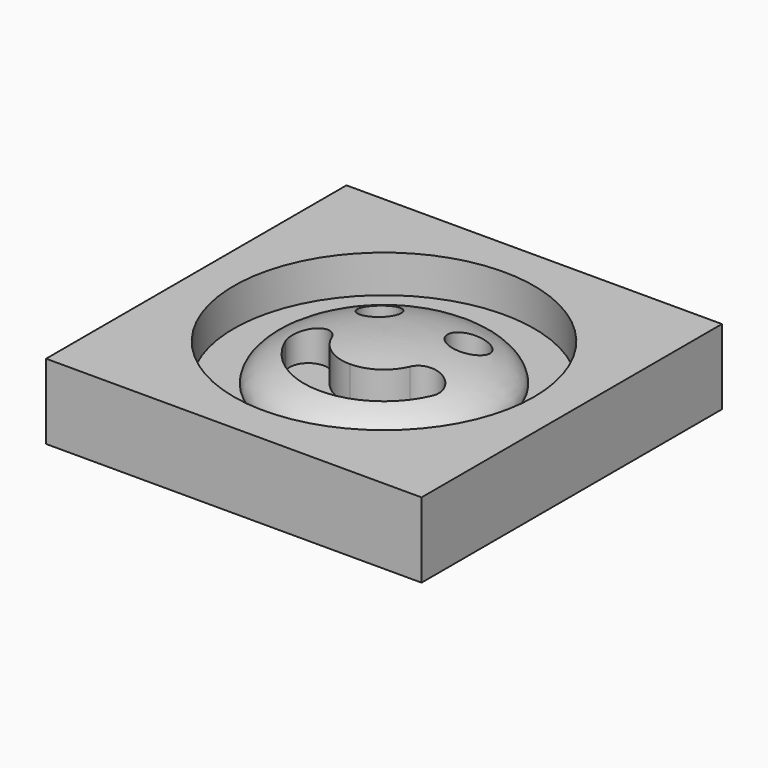
from build123d import *

# Parameters (mm, degrees)
F2_R     = 2.5
F3_DEPTH = 25
F4_R     = 20
F4_R_2   = 15
F4_R_3   = 2.5
F5_DEPTH = 5
F6_DEPTH = 5


with BuildPart() as f1:
    # F0 (on Front) → F1 (revolve)
    with BuildSketch(Plane.XZ):
        with BuildLine():
            Line((0, 0), (0, 5))
            add(Edge.make_bspline(
                [(0, 5), (-15, 5), (-15, 0)],
                knots=[4.7123889804, 4.7123889804, 4.7123889804, 6.2831853072, 6.2831853072, 6.2831853072], degree=2, weights=[1, 0.7071067812, 1]))
            Line((-15, 0), (0, 0))
        make_face()
    revolve(axis=Axis((0, 0, 2.5), (0, 0, 1)))

    # F2 (on face) → F3 (cut)
    with BuildSketch(Plane(origin=(0, 0, 0), x_dir=(1, 0, 0), z_dir=(0, 0, -1))):
        with Locations((5.9301354922, -6.6626928747)):
            Circle(F2_R)
        with BuildLine():
            ThreePointArc((-5.2131647244, 2.2031189874), (-3.1274667568, 4.7169663346), (0, 5.6595776977))
            ThreePointArc((0, 5.6595776977), (3.1274667568, 4.7169663346), (5.2131647244, 2.2031189874))
            ThreePointArc((5.2131647244, 2.2031189874), (8.4891528404, 0.8734942796), (9.8187775482, 4.1494823956))
            ThreePointArc((9.8187775482, 4.1494823956), (5.8904527284, 8.8842086506), (0, 10.6595776977))
            ThreePointArc((0, 10.6595776977), (-5.8904527284, 8.8842086506), (-9.8187775482, 4.1494823956))
            ThreePointArc((-9.8187775482, 4.1494823956), (-8.4891528404, 0.8734942796), (-5.2131647244, 2.2031189874))
        make_face()
        with Locations((-5.9301354922, -6.6626928747)):
            Circle(F2_R)
    extrude(amount=-F3_DEPTH, mode=Mode.SUBTRACT)

    # F4 (on face) → F5 (join)
    with BuildSketch(Plane(origin=(0, 0, 0), x_dir=(1, 0, 0), z_dir=(0, 0, -1))):
        Polygon((-25, -25), (0, -25), (25, -25), (25, 0), (25, 25), (0, 25), (-25, 25), (-25, 0), align=None)
        Circle(F4_R, mode=Mode.SUBTRACT)
        Circle(F4_R)
        Circle(F4_R_2, mode=Mode.SUBTRACT)
        Circle(F4_R_2)
        with Locations((-5.9301354922, -6.6626928747)):
            Circle(F4_R_3, mode=Mode.SUBTRACT)
        with Locations((5.9301354922, -6.6626928747)):
            Circle(F4_R_3, mode=Mode.SUBTRACT)
        with BuildLine():
            ThreePointArc((-5.2131647244, 2.2031189874), (-8.4891528404, 0.8734942796), (-9.8187775482, 4.1494823956))
            ThreePointArc((-9.8187775482, 4.1494823956), (0, 10.6595776977), (9.8187775482, 4.1494823956))
            ThreePointArc((9.8187775482, 4.1494823956), (8.4891528404, 0.8734942796), (5.2131647244, 2.2031189874))
            ThreePointArc((5.2131647244, 2.2031189874), (0, 5.6595776977), (-5.2131647244, 2.2031189874))
        make_face(mode=Mode.SUBTRACT)
        with BuildLine():
            ThreePointArc((9.8187775482, 4.1494823956), (0, 10.6595776977), (-9.8187775482, 4.1494823956))
            ThreePointArc((-9.8187775482, 4.1494823956), (-8.4891528404, 0.8734942796), (-5.2131647244, 2.2031189874))
            ThreePointArc((-5.2131647244, 2.2031189874), (0, 5.6595776977), (5.2131647244, 2.2031189874))
            ThreePointArc((5.2131647244, 2.2031189874), (8.4891528404, 0.8734942796), (9.8187775482, 4.1494823956))
        make_face()
        with Locations((5.9301354922, -6.6626928747)):
            Circle(F4_R_3)
        with Locations((-5.9301354922, -6.6626928747)):
            Circle(F4_R_3)
    extrude(amount=F5_DEPTH)

    # F4 (on face) → F6 (join)
    with BuildSketch(Plane(origin=(0, 0, 0), x_dir=(1, 0, 0), z_dir=(0, 0, -1))):
        Polygon((-25, -25), (0, -25), (25, -25), (25, 0), (25, 25), (0, 25), (-25, 25), (-25, 0), align=None)
        Circle(F4_R, mode=Mode.SUBTRACT)
    extrude(amount=-F6_DEPTH)


solid = f1.part
